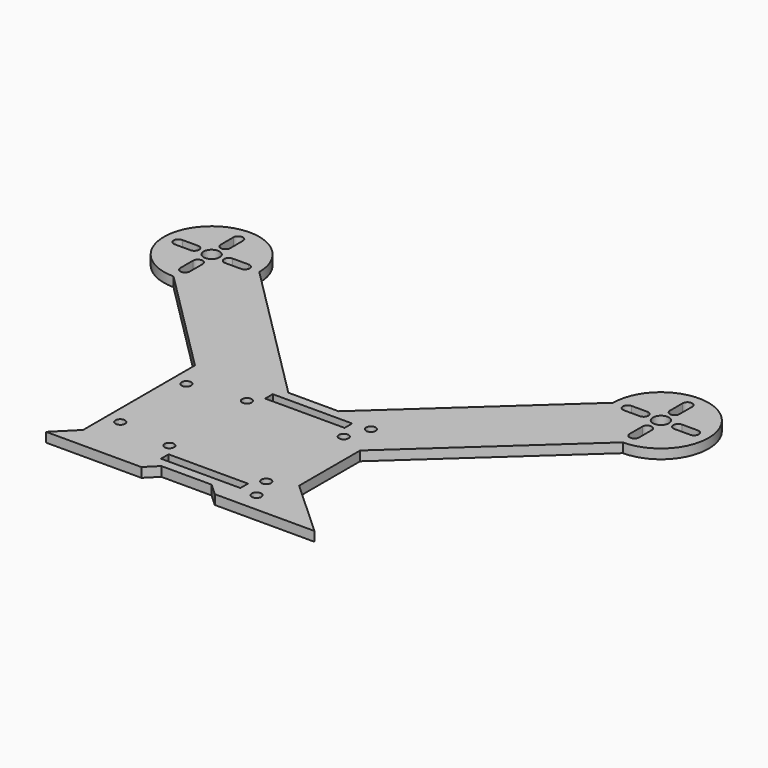
from build123d import *

# Parameters (mm, degrees)
F0_R     = 1.5
F0_W     = 25
F0_H     = 3
F0_R_2   = 2.5
F1_DEPTH = 3


# Not quite as in the source:
# - ends of sketch curves that miss each other by under 0.0002 mm in the source are joined


with BuildPart() as f1:
    # F0 (on Top) → F1 (new body)
    with BuildSketch(Plane.XY):
        with BuildLine():
            Line((-10.0000000587, 25), (-55.7106781187, 70.7106779065))
            ThreePointArc((-55.7106781187, 70.7106779065), (-81.3172799026, 81.3172797703), (-70.7106779065, 55.7106781187))
            Line((-70.7106779065, 55.7106781187), (-37, 22.0000003253))
            Line((-37, 22.0000003253), (-37, -22.0000003253))
            Line((-37, -22.0000003253), (-43.4767450368, -28.4767453404))
            Line((-43.4767450368, -28.4767453404), (-13.4767454108, -28.4767453404))
            Line((-13.4767454108, -28.4767453404), (-10.0000000587, -25))
            Line((-10.0000000587, -25), (5.8262266936, -25))
            Line((5.8262266936, -25), (9.6204284269, -28.4767453404))
            Line((9.6204284269, -28.4767453404), (40.9900556349, -28.4767453404))
            Line((40.9900556349, -28.4767453404), (23, -11.9918965954))
            Line((23, -11.9918965954), (23, 11.9918965954))
            Line((23, 11.9918965954), (70.7106780935, 55.7106781187))
            ThreePointArc((70.7106780935, 55.7106781187), (81.3172798365, 81.3172798365), (55.7106781187, 70.7106779065))
            Line((55.7106781187, 70.7106779065), (5.8262266936, 25))
            Line((5.8262266936, 25), (-10.0000000587, 25))
        make_face()
        with Locations((-15.25, -15.25)):
            Circle(F0_R, mode=Mode.SUBTRACT)
        with Locations((-32.5, -13)):
            Circle(F0_R, mode=Mode.SUBTRACT)
        with Locations((-32.5, 13)):
            Circle(F0_R, mode=Mode.SUBTRACT)
        with Locations((-15.25, 15.25)):
            Circle(F0_R, mode=Mode.SUBTRACT)
        with Locations((18, -22.5)):
            Circle(F0_R, mode=Mode.SUBTRACT)
        with Locations((0, -20.5)):
            Rectangle(F0_W, F0_H, mode=Mode.SUBTRACT)
        with Locations((15.25, -15.25)):
            Circle(F0_R, mode=Mode.SUBTRACT)
        with Locations((0, 20.5)):
            Rectangle(F0_W, F0_H, mode=Mode.SUBTRACT)
        with Locations((15.25, 15.25)):
            Circle(F0_R, mode=Mode.SUBTRACT)
        with Locations((18, 22.5)):
            Circle(F0_R, mode=Mode.SUBTRACT)
        with BuildLine():
            ThreePointArc((-72.2106780183, 65.2703154499), (-70.7106780132, 66.7703154448), (-69.2106780183, 65.2703154398))
            Line((-69.2106780183, 65.2703154398), (-69.210678035, 60.2703154398))
            ThreePointArc((-69.210678035, 60.2703154398), (-70.7106780401, 58.7703154448), (-72.210678035, 60.2703154499))
            Line((-72.210678035, 60.2703154499), (-72.2106780183, 65.2703154499))
        make_face(mode=Mode.SUBTRACT)
        with BuildLine():
            ThreePointArc((-76.1510407975, 72.2106782191), (-74.6510407925, 70.7106782241), (-76.1510407874, 69.2106782191))
            Line((-76.1510407874, 69.2106782191), (-81.1510407874, 69.2106782023))
            ThreePointArc((-81.1510407874, 69.2106782023), (-82.6510407925, 70.7106781972), (-81.1510407975, 72.2106782023))
            Line((-81.1510407975, 72.2106782023), (-76.1510407975, 72.2106782191))
        make_face(mode=Mode.SUBTRACT)
        with BuildLine():
            ThreePointArc((-68.9429111657, 72.4784450716), (-68.4009792874, 71.6673866996), (-68.2106781187, 70.7106781187))
            ThreePointArc((-68.2106781187, 70.7106781187), (-69.7539695377, 68.4009792874), (-72.4784450716, 68.9429111657))
            ThreePointArc((-72.4784450716, 68.9429111657), (-72.4784450716, 72.4784450716), (-68.9429111657, 72.4784450716))
        make_face(mode=Mode.SUBTRACT)
        with BuildLine():
            Line((-60.2703154398, 69.210678035), (-65.2703154398, 69.2106780183))
            ThreePointArc((-65.2703154398, 69.2106780183), (-66.7703154448, 70.7106780132), (-65.2703154499, 72.2106780183))
            Line((-65.2703154499, 72.2106780183), (-60.2703154499, 72.210678035))
            ThreePointArc((-60.2703154499, 72.210678035), (-58.7703154448, 70.7106780401), (-60.2703154398, 69.210678035))
        make_face(mode=Mode.SUBTRACT)
        with BuildLine():
            Line((-69.210678, 81.1510407925), (-69.210678, 76.1510407925))
            ThreePointArc((-69.210678, 76.1510407925), (-70.710678, 74.6510407925), (-72.210678, 76.1510407925))
            Line((-72.210678, 76.1510407925), (-72.210678, 81.1510407925))
            ThreePointArc((-72.210678, 81.1510407925), (-70.710678, 82.6510407925), (-69.210678, 81.1510407925))
        make_face(mode=Mode.SUBTRACT)
        with BuildLine():
            ThreePointArc((65.2703154499, 72.2106780183), (66.7703154448, 70.7106780132), (65.2703154398, 69.2106780183))
            Line((65.2703154398, 69.2106780183), (60.2703154398, 69.210678035))
            ThreePointArc((60.2703154398, 69.210678035), (58.7703154448, 70.7106780401), (60.2703154499, 72.210678035))
            Line((60.2703154499, 72.210678035), (65.2703154499, 72.2106780183))
        make_face(mode=Mode.SUBTRACT)
        with BuildLine():
            Line((69.210678035, 60.2703154398), (69.2106780183, 65.2703154398))
            ThreePointArc((69.2106780183, 65.2703154398), (70.7106780132, 66.7703154448), (72.2106780183, 65.2703154499))
            Line((72.2106780183, 65.2703154499), (72.210678035, 60.2703154499))
            ThreePointArc((72.210678035, 60.2703154499), (70.7106780401, 58.7703154448), (69.210678035, 60.2703154398))
        make_face(mode=Mode.SUBTRACT)
        with Locations((70.7106781187, 70.7106781187)):
            Circle(F0_R_2, mode=Mode.SUBTRACT)
        with BuildLine():
            Line((81.1510407874, 69.2106782023), (76.1510407874, 69.2106782191))
            ThreePointArc((76.1510407874, 69.2106782191), (74.6510407925, 70.7106782241), (76.1510407975, 72.2106782191))
            Line((76.1510407975, 72.2106782191), (81.1510407975, 72.2106782023))
            ThreePointArc((81.1510407975, 72.2106782023), (82.6510407925, 70.7106781972), (81.1510407874, 69.2106782023))
        make_face(mode=Mode.SUBTRACT)
        with BuildLine():
            Line((72.210678, 81.1510407925), (72.210678, 76.1510407925))
            ThreePointArc((72.210678, 76.1510407925), (70.710678, 74.6510407925), (69.210678, 76.1510407925))
            Line((69.210678, 76.1510407925), (69.210678, 81.1510407925))
            ThreePointArc((69.210678, 81.1510407925), (70.710678, 82.6510407925), (72.210678, 81.1510407925))
        make_face(mode=Mode.SUBTRACT)
    extrude(amount=F1_DEPTH)


solid = f1.part
